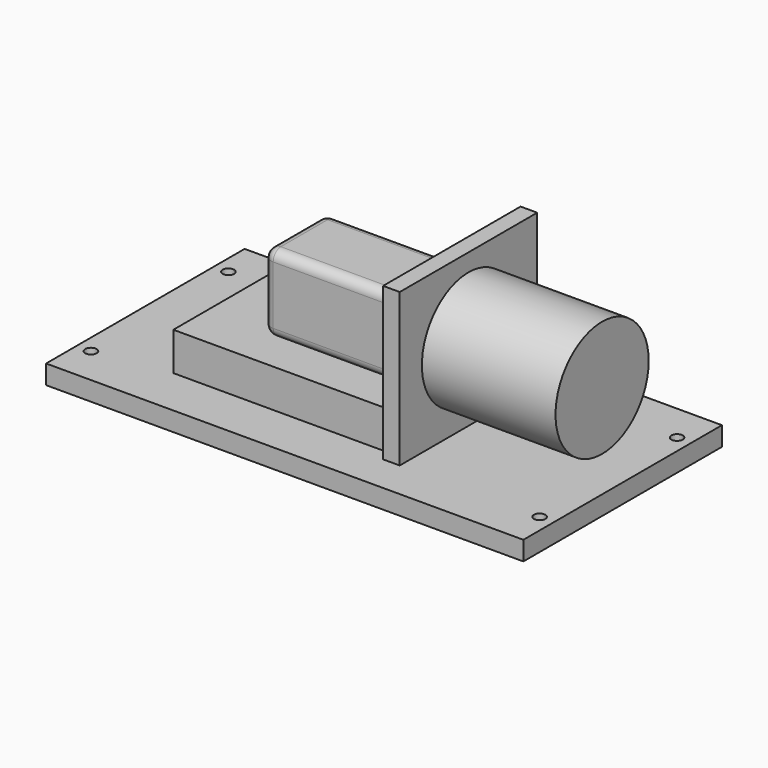
from build123d import *

# Parameters (mm, degrees)
F0_W     = 250
F0_H     = 130
F0_R     = 3
F1_DEPTH = 10
F2_W     = 114.71279338
F2_H     = 77.8716804087
F2_R     = 2.75
F3_DEPTH = 20
F4_DEPTH = 80
F6_W     = 0.0666481256
F6_H     = 40.6
F6_W_2   = 69.9333518744
F7_DEPTH = 40.6
F8_R     = 5
F9_DEPTH = 70


with BuildPart() as f1:
    # F0 (on Top) → F1 (new body)
    with BuildSketch(Plane.XY):
        with Locations((125, 65)):
            Rectangle(F0_W, F0_H)
        with Locations((7.5, 20)):
            Circle(F0_R, mode=Mode.SUBTRACT)
        with Locations((242.5, 20)):
            Circle(F0_R, mode=Mode.SUBTRACT)
        with Locations((7.5, 110)):
            Circle(F0_R, mode=Mode.SUBTRACT)
        with Locations((242.5, 110)):
            Circle(F0_R, mode=Mode.SUBTRACT)
    extrude(amount=-F1_DEPTH)


with BuildPart() as f3:
    # F2 (on Top) → F3 (new body)
    with BuildSketch(Plane.XY):
        with Locations((103.3462490886, 64.7845622897)):
            Rectangle(F2_W, F2_H)
        with Locations((152.6860141896, 64.9501949326)):
            Circle(F2_R, mode=Mode.SUBTRACT)
        Polygon((160.7026457787, 109.7845622897), (160.7026457787, 103.7204024941), (160.7026457787, 25.8487220854), (160.7026457787, 19.7845622897), (169.4147884846, 19.7845622897), (169.4147884846, 109.7845622897), align=None)
    extrude(amount=F3_DEPTH)


with BuildPart() as f4:
    # F2 (on Top) → F4 (new body)
    with BuildSketch(Plane.XY):
        Polygon((160.7026457787, 109.7845622897), (160.7026457787, 103.7204024941), (160.7026457787, 25.8487220854), (160.7026457787, 19.7845622897), (169.4147884846, 19.7845622897), (169.4147884846, 109.7845622897), align=None)
    extrude(amount=F4_DEPTH)

    # F5 (on face) → F9 (join)
    with BuildSketch(Plane.YZ.offset(169.4147884846)):
        with BuildLine():
            ThreePointArc((95.2830868442, 40), (95.2841934261, 40.1499981859), (95.2845622897, 40.3))
            ThreePointArc((95.2845622897, 40.3), (64.6345604756, 70.7996311364), (34.2860377352, 40))
            ThreePointArc((34.2860377352, 40), (64.7845622897, 9.8), (95.2830868442, 40))
        make_face()
    extrude(amount=F9_DEPTH)


with BuildPart() as f7:
    # F6 (on face) → F7 (new body)
    with BuildSketch(Plane.XY.offset(20)):
        with Locations((148.0660647154, 65.1399716735)):
            Rectangle(F6_W, F6_H)
        with Locations((113.0660647154, 65.1399716735)):
            Rectangle(F6_W_2, F6_H)
    extrude(amount=F7_DEPTH)

    # F8
    f8_edges = [f7.edges().sort_by_distance(p)[0] for p in [
        (78.099389, 65.139972, 60.6),
        (113.099389, 85.439972, 60.6),
        (113.099389, 44.839972, 60.6),
        (148.099389, 65.139972, 60.6),
        (148.099389, 44.839972, 40.3),
        (113.099389, 44.839972, 20),
        (78.099389, 44.839972, 40.3),
        (78.099389, 65.139972, 20),
        (78.099389, 85.439972, 40.3),
        (113.099389, 85.439972, 20),
        (148.099389, 85.439972, 40.3),
    ]]
    fillet(f8_edges, radius=F8_R)


solid = Compound([f1.part, f3.part, f4.part, f7.part])
